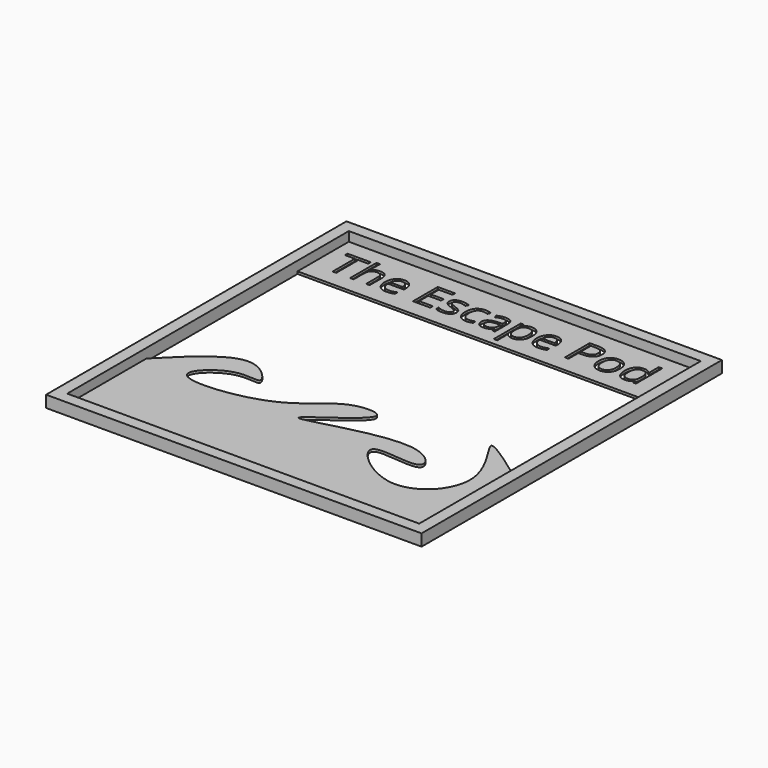
from build123d import *

# Parameters (mm, degrees)
F0_W         = 101.6
F0_H         = 101.6
F1_DEPTH     = 3.175
F2_W         = 95.25
F2_H         = 95.25
F3_DEPTH     = 2.54
F5_DEPTH     = 25.4
F6_TEXT_SIZE = 11.7515110307
F7_DEPTH     = 2.54


# Not quite as in the source:
# - the program builds the solid bodies; features that only make, move or delete a surface that nothing else refers to are left out
# - Text() gives the source's letters only with a copy of the font that has no kerning and outlines rounded to 1/6400 em; it was checked with that copy


with BuildPart() as f1:
    # F0 (on Top) → F1 (new body)
    with BuildSketch(Plane.XY):
        with Locations((-3.5059135407, 0.2663029191)):
            Rectangle(F0_W, F0_H)
    extrude(amount=F1_DEPTH)

    # F2 (on face) → F3 (cut)
    with BuildSketch(Plane.XY.offset(3.175)):
        with Locations((-3.5059135407, 0.2663029191)):
            Rectangle(F2_W, F2_H)
    extrude(amount=-F3_DEPTH, mode=Mode.SUBTRACT)

    # F4 (on face) → F5 (cut)
    with BuildSketch(Plane.XY.offset(0.635)):
        with BuildLine():
            Line((-51.1309135407, 30.5515490472), (-51.1309135407, -20.5346476287))
            add(Edge.make_bspline(
                [(-51.1309135407, -20.5346476287), (-44.4772618326, -13.8302906183), (-33.9068828394, -3.179358226), (-23.2203086294, -15.3563460522), (-32.9684424192, -11.6092342173), (-47.3475791877, -24.5641943321), (-14.4462224349, -21.5999426076), (-6.9098977612, -8.6661607427), (9.795318715, -9.5482538946), (-23.6487982838, -28.8557073487), (18.759969453, -11.7235185907), (28.9023260409, -25.7167638479), (3.8784186559, -18.7465846699), (25.9933819087, -39.1418427373), (42.8977648414, -21.3805820295), (24.3405359568, -0.4179396645), (37.5035789914, -9.9728197395), (44.1190864593, -14.7749297321)],
                knots=[0, 0, 0, 0, 0.0843868265, 0.1340618321, 0.1785698343, 0.2355024324, 0.3184971147, 0.3922127471, 0.43864444, 0.5100413192, 0.6038049761, 0.653403458, 0.7150039849, 0.785434313, 0.8590406783, 0.9291563932, 1, 1, 1, 1], degree=3))
            Line((44.1190864593, -14.7749297321), (44.1190864593, 30.5515490472))
            Line((44.1190864593, 30.5515490472), (-51.1309135407, 30.5515490472))
        make_face()
    extrude(amount=-F5_DEPTH, mode=Mode.SUBTRACT)

    # F6 (on face) → F7 (cut)
    with BuildSketch(Plane.XY.offset(0.635)):
        with Locations((-48.0388700962, 35.0815467536)):
            Text('The Escape Pod', F6_TEXT_SIZE, font='Open Sans', text_align=(TextAlign.LEFT, TextAlign.BOTTOM))
    extrude(amount=-F7_DEPTH, mode=Mode.SUBTRACT)


solid = f1.part
